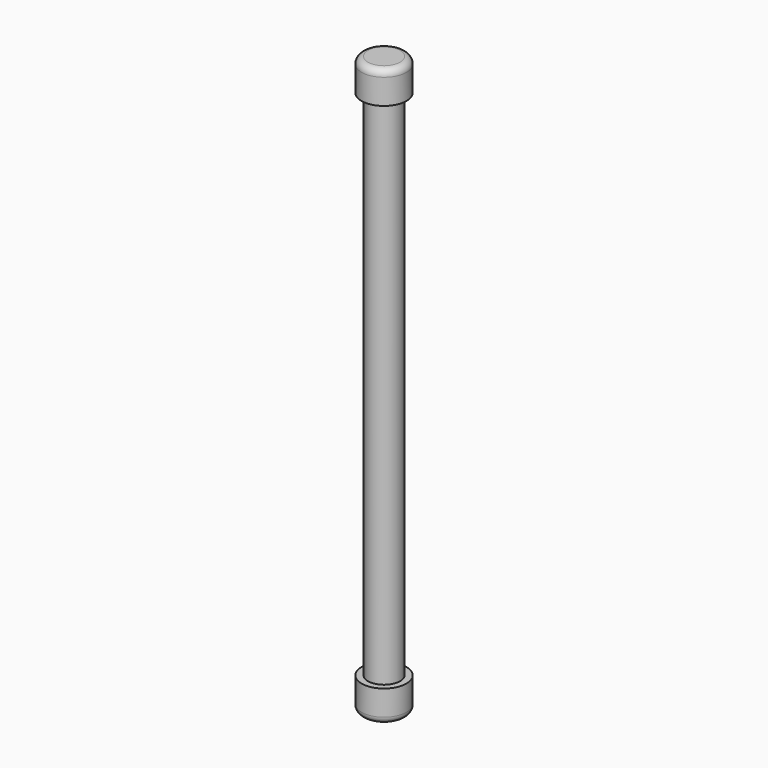
from build123d import *

# Parameters (mm, degrees)
F0_R     = 3.33375
F0_R_2   = 2.38125
F1_DEPTH = 4.7625
F3_R     = 2.38125
F4_DEPTH = 4.7625
F5_DEPTH = 80.9625
F6_R     = 3.33375
F7_DEPTH = 4.7625
F8_R     = 1.016


# Not quite as in the source:
# - a fillet or chamfer that OpenCascade refuses, or shapes differently, is made with other operations: its cross-section is extruded or revolved along the edge and cut away or added


with BuildPart() as f1:
    # F0 (on Top) → F1 (new body)
    with BuildSketch(Plane.XY):
        Circle(F0_R)
        Circle(F0_R_2, mode=Mode.SUBTRACT)
    extrude(amount=F1_DEPTH)

    # F2: fillet of radius 1.016 on 1 edges, made by hand

    # F2_s1 → F2_t2 (revolve, cut)
    with BuildSketch(Plane.XZ):
        with BuildLine():
            ThreePointArc((3.33375, 3.7484863167), (3.0582808906, 4.4440939647), (2.38125, 4.7625))
            Line((2.38125, 4.7625), (3.33375, 4.7625))
            Line((3.33375, 4.7625), (3.33375, 3.7484863167))
        make_face()
    revolve(axis=Axis((0, 0, 4.7625), (0, 0, 1)), mode=Mode.SUBTRACT)

    # F3 (on Top) → F4 (join)
    with BuildSketch(Plane.XY):
        Circle(F3_R)
    extrude(amount=F4_DEPTH)

    # F3 (on Top) → F5 (join)
    with BuildSketch(Plane.XY):
        Circle(F3_R)
    extrude(amount=-F5_DEPTH)

    # F6 (on face) → F7 (join)
    with BuildSketch(Plane(origin=(0, 0, -80.9625), x_dir=(1, 0, 0), z_dir=(0, 0, -1))):
        Circle(F6_R)
    extrude(amount=-F7_DEPTH)

    # F8
    f8_edges = [f1.edges().sort_by_distance(p)[0] for p in [
        (-3.33375, 0, -80.9625),
    ]]
    fillet(f8_edges, radius=F8_R)


solid = f1.part
